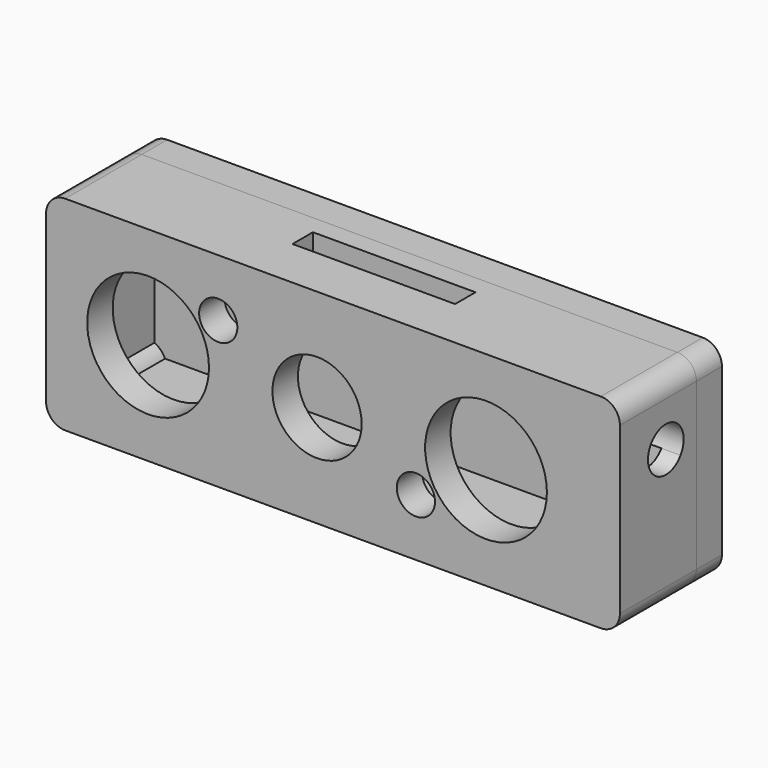
from build123d import *

# Parameters (mm, degrees)
F0_R      = 1.25
F1_DEPTH  = 5
F2_R      = 1.25
F3_DEPTH  = 10
F4_R      = 3
F4_R_2    = 9.55
F4_R_3    = 7
F5_DEPTH  = 5
F6_W      = 25.5
F6_H      = 4
F7_DEPTH  = 5
F8_R      = 3
F8_2_R    = 3
F10_DEPTH = 10
F11_DEPTH = 7
F12_D     = 5.1


# Not quite as in the source:
# - a feature names something its author has since deleted; it is built from what else it names


with BuildPart() as f1:
    # F0 (on Front) → F1 (new body)
    with BuildSketch(Plane.XZ):
        Polygon((47.5, 16), (42.5, 16), (-42.5, 16), (-42.5, -16), (42.5, -16), (47.5, -16), align=None)
        with Locations((-39, -12.5)):
            Circle(F0_R, mode=Mode.SUBTRACT)
        with Locations((44, -12.5)):
            Circle(F0_R, mode=Mode.SUBTRACT)
        with Locations((-39, 12.5)):
            Circle(F0_R, mode=Mode.SUBTRACT)
        with Locations((44, 12.5)):
            Circle(F0_R, mode=Mode.SUBTRACT)
    extrude(amount=F1_DEPTH)

    # F8#2
    f8_2_edges = [f1.edges().sort_by_distance(p)[0] for p in [
        (47.5, -2.5, 16),
        (47.5, -2.5, -16),
        (-42.5, -2.5, 16),
        (-42.5, -2.5, -16),
    ]]
    fillet(f8_2_edges, radius=F8_2_R)


with BuildPart() as f3:
    # F2 (on face) → F3 (new body)
    with BuildSketch(Plane.XZ.offset(5)):
        with BuildLine():
            ThreePointArc((-37.5, 9.3377223398), (-40.8708286934, 9.5419601085), (-42.5, 12.5))
            Line((-42.5, 12.5), (-42.5, -12.5))
            ThreePointArc((-42.5, -12.5), (-40.8708286934, -9.5419601085), (-37.5, -9.3377223398))
            Line((-37.5, -9.3377223398), (-37.5, 9.3377223398))
        make_face()
        with BuildLine():
            ThreePointArc((-35.5, 12.5), (-36.5251262658, 14.9748737342), (-39, 16))
            ThreePointArc((-39, 16), (-41.4748737342, 14.9748737342), (-42.5, 12.5))
            ThreePointArc((-42.5, 12.5), (-40.8708286934, 9.5419601085), (-37.5, 9.3377223398))
            Line((-37.5, 9.3377223398), (-37.5, 11))
            Line((-37.5, 11), (-35.8377223398, 11))
            ThreePointArc((-35.8377223398, 11), (-35.5854742781, 11.7312255892), (-35.5, 12.5))
        make_face()
        with Locations((-39, 12.5)):
            Circle(F2_R, mode=Mode.SUBTRACT)
        with BuildLine():
            Line((-39, 16), (-42.5, 16))
            Line((-42.5, 16), (-42.5, 12.5))
            ThreePointArc((-42.5, 12.5), (-41.4748737342, 14.9748737342), (-39, 16))
        make_face()
        with BuildLine():
            ThreePointArc((-39, -16), (-41.4748737342, -14.9748737342), (-42.5, -12.5))
            Line((-42.5, -12.5), (-42.5, -16))
            Line((-42.5, -16), (-39, -16))
        make_face()
        with BuildLine():
            ThreePointArc((-37.5, -9.3377223398), (-40.8708286934, -9.5419601085), (-42.5, -12.5))
            ThreePointArc((-42.5, -12.5), (-41.4748737342, -14.9748737342), (-39, -16))
            ThreePointArc((-39, -16), (-36.5251262658, -14.9748737342), (-35.5, -12.5))
            ThreePointArc((-35.5, -12.5), (-35.5854742781, -11.7312255892), (-35.8377223398, -11))
            Line((-35.8377223398, -11), (-37.5, -11))
            Line((-37.5, -11), (-37.5, -9.3377223398))
        make_face()
        with Locations((-39, -12.5)):
            Circle(F2_R, mode=Mode.SUBTRACT)
        with BuildLine():
            Line((42.5, 16), (-39, 16))
            ThreePointArc((-39, 16), (-36.5251262658, 14.9748737342), (-35.5, 12.5))
            ThreePointArc((-35.5, 12.5), (-35.5854742781, 11.7312255892), (-35.8377223398, 11))
            Line((-35.8377223398, 11), (37.5, 11))
            Line((37.5, 11), (37.5, -11))
            Line((37.5, -11), (-35.8377223398, -11))
            ThreePointArc((-35.8377223398, -11), (-35.5854742781, -11.7312255892), (-35.5, -12.5))
            ThreePointArc((-35.5, -12.5), (-36.5251262658, -14.9748737342), (-39, -16))
            Line((-39, -16), (42.5, -16))
            Line((42.5, -16), (47.5, -16))
            Line((47.5, -16), (47.5, 16))
            Line((47.5, 16), (42.5, 16))
        make_face()
        with Locations((44, -12.5)):
            Circle(F2_R, mode=Mode.SUBTRACT)
        with Locations((44, 12.5)):
            Circle(F2_R, mode=Mode.SUBTRACT)
        with BuildLine():
            Line((-37.5, 11), (-37.5, 9.3377223398))
            ThreePointArc((-37.5, 9.3377223398), (-36.5251262658, 10.0251262658), (-35.8377223398, 11))
            Line((-35.8377223398, 11), (-37.5, 11))
        make_face()
        with BuildLine():
            ThreePointArc((-35.8377223398, -11), (-36.5251262658, -10.0251262658), (-37.5, -9.3377223398))
            Line((-37.5, -9.3377223398), (-37.5, -11))
            Line((-37.5, -11), (-35.8377223398, -11))
        make_face()
    extrude(amount=F3_DEPTH)

    # F4 (on face) → F5 (join)
    with BuildSketch(Plane.XZ.offset(15)):
        Polygon((42.5, 16), (-42.5, 16), (-42.5, -16), (42.5, -16), (47.5, -16), (47.5, 16), align=None)
        with Locations((15.5, -7)):
            Circle(F4_R, mode=Mode.SUBTRACT)
        with Locations((-26.5, 0)):
            Circle(F4_R_2, mode=Mode.SUBTRACT)
        Circle(F4_R_3, mode=Mode.SUBTRACT)
        with Locations((-15.5, 7)):
            Circle(F4_R, mode=Mode.SUBTRACT)
        with Locations((26.5, 0)):
            Circle(F4_R_2, mode=Mode.SUBTRACT)
    extrude(amount=F5_DEPTH)

    # F6 (on face) → F7 (cut)
    with BuildSketch(Plane.XY.offset(16)):
        with Locations((2.5, -10)):
            Rectangle(F6_W, F6_H)
    extrude(amount=-F7_DEPTH, mode=Mode.SUBTRACT)

    # F8
    f8_edges = [f3.edges().sort_by_distance(p)[0] for p in [
        (47.5, -12.5, 16),
        (47.5, -12.5, -16),
        (-42.5, -12.5, 16),
        (-42.5, -12.5, -16),
    ]]
    fillet(f8_edges, radius=F8_R)

    # F9 (on face) → F10 (cut, through all)
    with BuildSketch(Plane(origin=(37.5, 0, 0), x_dir=(0, -1, 0), z_dir=(-1, 0, 0))):
        with BuildLine():
            ThreePointArc((13.8844104576, 4.0175327715), (14.3425616376, 4.9620781825), (14.5, 6))
            ThreePointArc((14.5, 6), (9.9620781825, 9.3425616376), (8.1155895424, 4.0175327715))
            ThreePointArc((8.1155895424, 4.0175327715), (11, 2.5), (13.8844104576, 4.0175327715))
        make_face()
    extrude(amount=-F10_DEPTH, mode=Mode.SUBTRACT)

    # F9 (on face) → F11 (cut)
    with BuildSketch(Plane(origin=(37.5, 0, 0), x_dir=(0, -1, 0), z_dir=(-1, 0, 0))):
        with BuildLine():
            ThreePointArc((13.8844104576, 4.0175327715), (14.3425616376, 4.9620781825), (14.5, 6))
            ThreePointArc((14.5, 6), (9.9620781825, 9.3425616376), (8.1155895424, 4.0175327715))
            ThreePointArc((8.1155895424, 4.0175327715), (11, 2.5), (13.8844104576, 4.0175327715))
        make_face()
        with BuildLine():
            ThreePointArc((13.8844104576, 4.0175327715), (11, 2.5), (8.1155895424, 4.0175327715))
            Line((8.1155895424, 4.0175327715), (9.1571289137, -7.8122533804))
            ThreePointArc((9.1571289137, -7.8122533804), (10.9187950419, -5.8017830877), (12.85, -7.65))
            ThreePointArc((12.85, -7.65), (12.8482169123, -7.7312049581), (12.8428710863, -7.8122533804))
            Line((12.8428710863, -7.8122533804), (13.8844104576, 4.0175327715))
        make_face()
        with BuildLine():
            Line((12.8428710863, -7.8122533804), (9.1571289137, -7.8122533804))
            ThreePointArc((9.1571289137, -7.8122533804), (11, -9.5), (12.8428710863, -7.8122533804))
        make_face()
        with BuildLine():
            ThreePointArc((12.85, -7.65), (10.9187950419, -5.8017830877), (9.1571289137, -7.8122533804))
            Line((9.1571289137, -7.8122533804), (12.8428710863, -7.8122533804))
            ThreePointArc((12.8428710863, -7.8122533804), (12.8482169123, -7.7312049581), (12.85, -7.65))
        make_face()
    extrude(amount=-F11_DEPTH, mode=Mode.SUBTRACT)

    # F12 (through all)
    with Locations(Plane(origin=(37.5, 0, 0), x_dir=(0, -1, 0), z_dir=(1, 0, 0))):
        with Locations((11, -6)):
            Hole(F12_D / 2)


solid = Compound([f1.part, f3.part])
